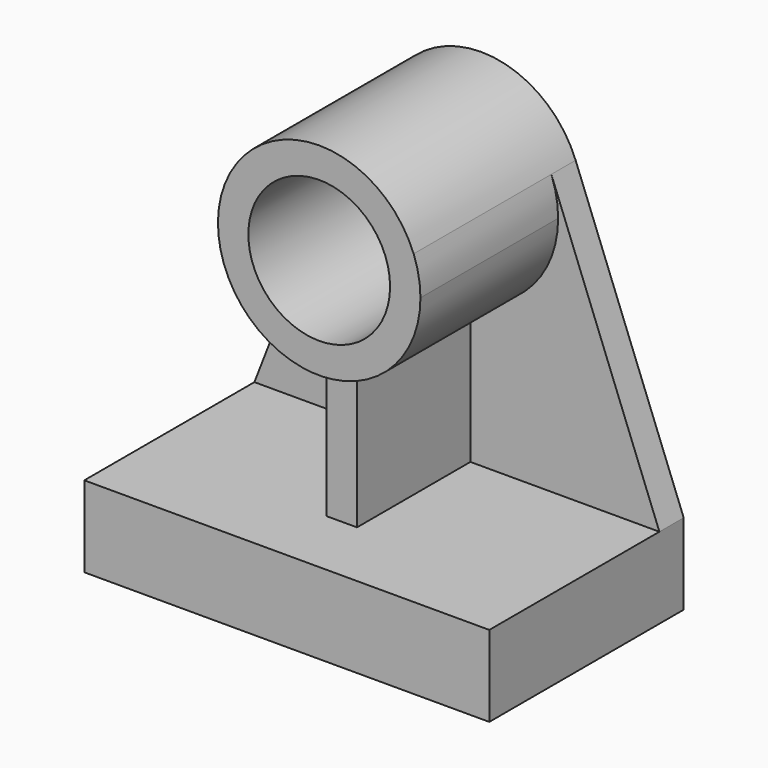
from build123d import *

# Parameters (mm, degrees)
F2_DEPTH = 107.95
F3_DEPTH = 152.4
F4_DEPTH = 19.05
F1_R     = 44.45
F5_DEPTH = 127


# Not quite as in the source:
# - a variable given as a bare number and used for a length is read in inches; the dataset says mm whatever the document's units were


with BuildPart() as f2:
    # F1 (on Front) → F2 (new body)
    with BuildSketch(Plane.XZ):
        with BuildLine():
            Line((-10.5833333333, 115.1881556289), (-10.5833333333, 25.4))
            Line((-10.5833333333, 25.4), (8.4666666667, 25.4))
            Line((8.4666666667, 25.4), (8.4666666667, 114.8669756364))
            ThreePointArc((8.4666666667, 114.8669756364), (-1.0704478462, 114.3090231497), (-10.5833333333, 115.1881556289))
        make_face()
    extrude(amount=F2_DEPTH)

    # F1 (on Front) → F3 (join)
    with BuildSketch(Plane.XZ):
        Polygon((-10.5833333333, 25.4), (-127, 25.4), (-127, -25.4), (127, -25.4), (127, 25.4), (8.4666666667, 25.4), align=None)
    extrude(amount=F3_DEPTH)

    # F1 (on Front) → F4 (join)
    with BuildSketch(Plane.XZ):
        with BuildLine():
            Line((-59.2277468166, 200.6981223472), (-127, 25.4))
            Line((-127, 25.4), (-10.5833333333, 25.4))
            Line((-10.5833333333, 25.4), (-10.5833333333, 115.1881556289))
            ThreePointArc((-10.5833333333, 115.1881556289), (-55.1940696993, 146.4015180298), (-59.2277468166, 200.6981223472))
        make_face()
        with BuildLine():
            Line((8.4666666667, 114.8669756364), (8.4666666667, 25.4))
            Line((8.4666666667, 25.4), (127, 25.4))
            Line((127, 25.4), (59.2277468166, 200.6981223472))
            ThreePointArc((59.2277468166, 200.6981223472), (62.4228000127, 189.4466320699), (63.5, 177.8))
            ThreePointArc((63.5, 177.8), (47.801063447, 135.9991826236), (8.4666666667, 114.8669756364))
        make_face()
    extrude(amount=F4_DEPTH)

    # F1 (on Front) → F5 (join)
    with BuildSketch(Plane.XZ):
        with BuildLine():
            ThreePointArc((59.2277468166, 200.6981223472), (0, 241.3), (-59.2277468166, 200.6981223472))
            ThreePointArc((-59.2277468166, 200.6981223472), (-55.1940696993, 146.4015180298), (-10.5833333333, 115.1881556289))
            ThreePointArc((-10.5833333333, 115.1881556289), (-1.0704478462, 114.3090231497), (8.4666666667, 114.8669756364))
            ThreePointArc((8.4666666667, 114.8669756364), (47.801063447, 135.9991826236), (63.5, 177.8))
            ThreePointArc((63.5, 177.8), (62.4228000127, 189.4466320699), (59.2277468166, 200.6981223472))
        make_face()
        with Locations((0, 177.8)):
            Circle(F1_R, mode=Mode.SUBTRACT)
    extrude(amount=F5_DEPTH)


solid = f2.part
